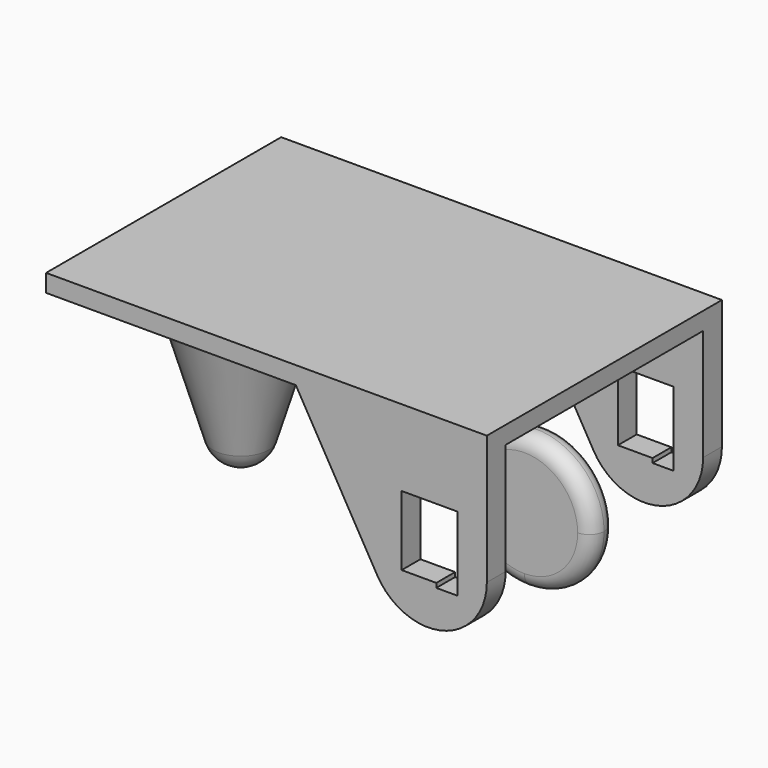
from build123d import *

# Parameters (mm, degrees)
F0_W     = 150
F0_H     = 100
F1_DEPTH = 6
F5_DEPTH = 100
F3_W     = 171.0709459866
F3_H     = 84
F6_DEPTH = 200
F8_DEPTH = 10
F9_R     = 4.99999


# Not quite as in the source:
# - a fillet or chamfer is up to 0.001 mm smaller than in the source, because OpenCascade refuses the exact size


with BuildPart() as f1:
    # F0 (on Top) → F1 (new body)
    with BuildSketch(Plane.XY):
        Rectangle(F0_W, F0_H)
    extrude(amount=F1_DEPTH)

    # F2 (on face) → F5 (join)
    with BuildSketch(Plane.XZ.offset(50)):
        with BuildLine():
            Line((75, 0), (10, 0))
            Line((10, 0), (37.6794919243, -47.9422863406))
            ThreePointArc((37.6794919243, -47.9422863406), (60.1763809021, -57.2608028664), (75, -37.9422863406))
            Line((75, -37.9422863406), (75, 0))
        make_face()
        Polygon((46, -20), (65, -20), (65, -45.2), (57.8, -45.2), (57.8, -43.7), (46, -43.7), align=None, mode=Mode.SUBTRACT)
    extrude(amount=-F5_DEPTH)

    # F3 (on Top) → F6 (cut)
    with BuildSketch(Plane.XY):
        with Locations((25.0738235191, 0)):
            Rectangle(F3_W, F3_H)
    extrude(amount=-F6_DEPTH, mode=Mode.SUBTRACT)

    # F4 (on Front) → F7 (revolve)
    with BuildSketch(Plane.XZ):
        with BuildLine():
            Line((-48.7436212599, 0), (-75, 0))
            Line((-75, 0), (-58.2256204143, -55.7750751688))
            ThreePointArc((-58.2256204143, -55.7750751688), (-58.2296045097, -50.0849254651), (-55.1008508317, -45.3321662722))
            Line((-55.1008508317, -45.3321662722), (-66.9300179817, -6))
            Line((-66.9300179817, -6), (-48.7436212599, -6))
            Line((-48.7436212599, -6), (-48.7436212599, 0))
        make_face()
        with BuildLine():
            ThreePointArc((-55.1008508317, -45.3321662722), (-58.2296045097, -50.0849254651), (-58.2256204143, -55.7750751688))
            ThreePointArc((-58.2256204143, -55.7750751688), (-54.6514212532, -60.8693328985), (-48.7436212599, -62.8249046049))
            Line((-48.7436212599, -62.8249046049), (-48.7436212599, -52.923359872))
            Line((-48.7436212599, -52.923359872), (-52.8177958548, -52.923359872))
            Line((-52.8177958548, -52.923359872), (-55.1008508317, -45.3321662722))
        make_face()
    revolve(axis=Axis((-48.7436212599, 0, -43.6514355242), (0, 0, -1)))


with BuildPart() as f8:
    # F4 (on Front) → F8 (new body)
    with BuildSketch(Plane.XZ):
        with BuildLine():
            ThreePointArc((78.8968328855, -39.7), (39.4201513826, -23.3482231771), (55.7719283868, -62.8249046049))
            ThreePointArc((55.7719283868, -62.8249046049), (72.1237051786, -56.0517768229), (78.8968328855, -39.7))
        make_face()
    extrude(amount=F8_DEPTH)

    # F9 (radius 5 in the source; OpenCascade refuses exactly that, so slightly less here)
    f9_edges = [f8.edges().sort_by_distance(p)[0] for p in [
        (55.771928, 0, -16.575095),
        (55.771928, -5, -62.824905),
        (55.771928, -10, -16.575095),
    ]]
    fillet(f9_edges, radius=F9_R)


solid = Compound([f1.part, f8.part])
